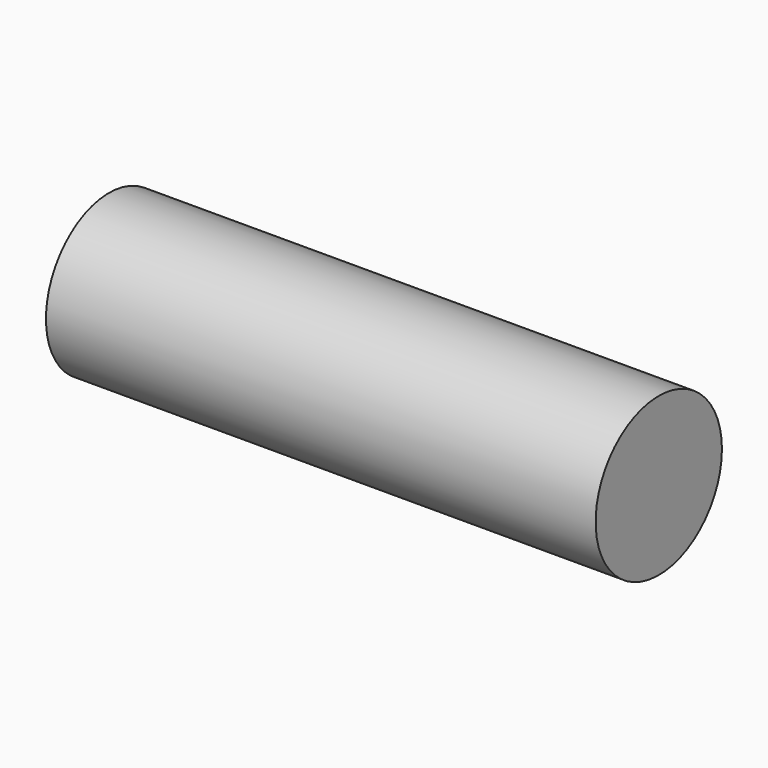
from build123d import *

# Parameters (mm, degrees)
F4_R     = 7.25
F5_DEPTH = 25.25


with BuildPart() as f5:
    # F4 (on Right) → F5 (new body, symmetric)
    with BuildSketch(Plane.YZ):
        with Locations((-5, 3)):
            Circle(F4_R)
    extrude(amount=F5_DEPTH, both=True)


solid = f5.part
